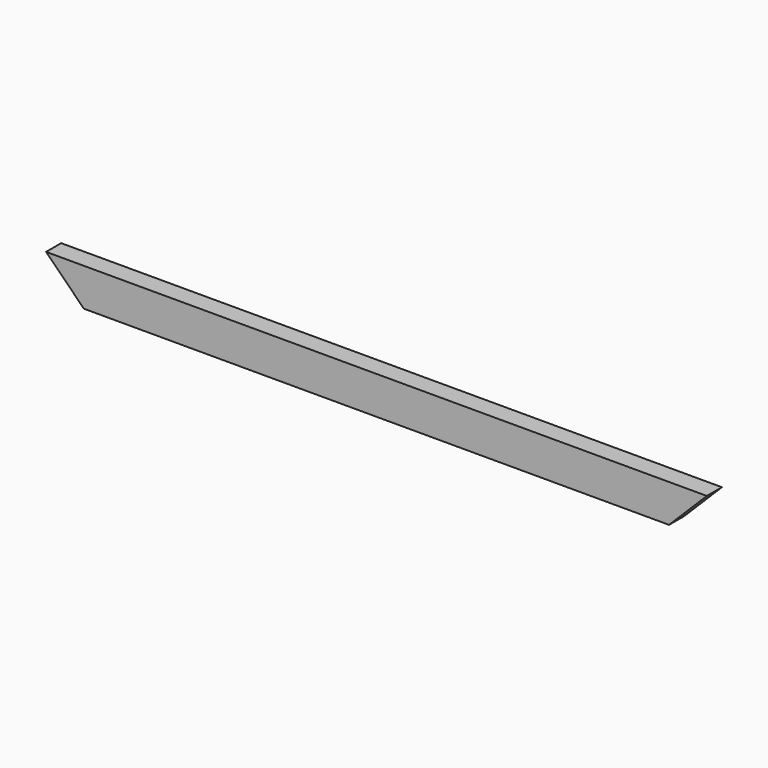
from build123d import *

# Parameters (mm, degrees)
F0_W     = 350
F0_H     = 20
F1_DEPTH = 10
F2_SIZE  = 19.99999


# Not quite as in the source:
# - a fillet or chamfer is up to 0.001 mm smaller than in the source, because OpenCascade refuses the exact size


with BuildPart() as f1:
    # F0 (on Front) → F1 (new body)
    with BuildSketch(Plane.XZ):
        with Locations((102.8835877776, 29.5569973439)):
            Rectangle(F0_W, F0_H)
    extrude(amount=F1_DEPTH)

    # F2 (size 20 in the source; OpenCascade refuses exactly that, so slightly less here)
    f2_edges = [f1.edges().sort_by_distance(p)[0] for p in [
        (-72.116412, -5, 19.556997),
        (277.883588, -5, 19.556997),
    ]]
    chamfer(f2_edges, length=F2_SIZE)


solid = f1.part
